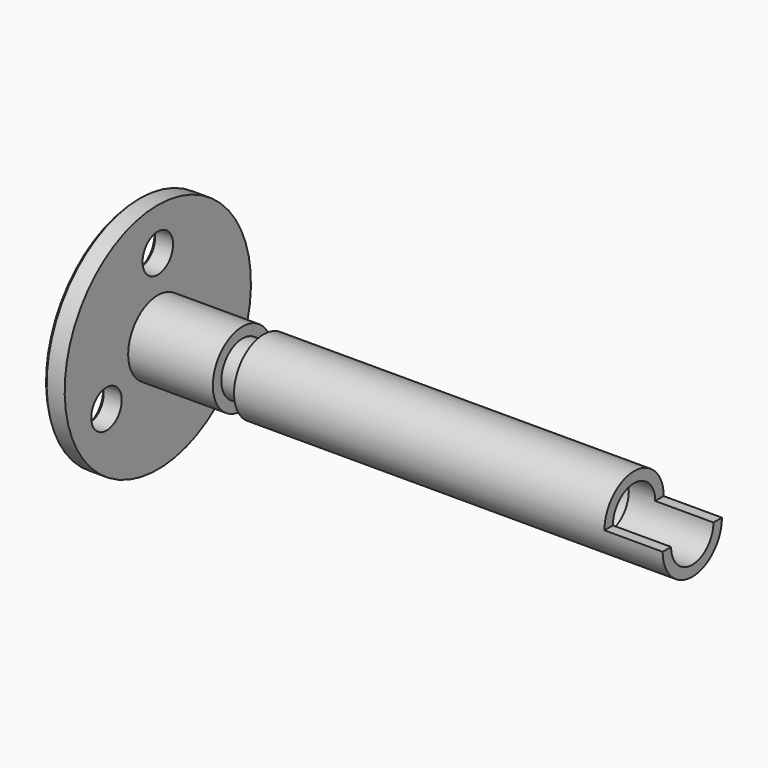
from build123d import *

# Parameters (mm, degrees)
F3_DEPTH        = 5.5
F5_D            = 3.6
F5_COPIES_COUNT = 3
F6_SIZE         = 0.3


# Not quite as in the source:
# - a pattern or mirror of a feature is missing from the dataset's text; its kind, count and spacing are read off the source's solid


with BuildPart() as f1:
    # F0 (on Front) → F1 (revolve)
    with BuildSketch(Plane.XZ):
        Polygon((0, 11), (0, 0), (42, 0), (44.5, 2.5), (52.5, 2.5), (52.5, 3.5), (12, 3.5), (12, 2.5), (10, 2.5), (10, 3.5), (2, 3.5), (2, 11), align=None)
    revolve(axis=Axis((21, 0, 0), (-1, 0, 0)))

    # F2 (on face) → F3 (cut)
    with BuildSketch(Plane.YZ.offset(52.5)):
        with BuildLine():
            Line((2.5, 0), (3.5, 0))
            ThreePointArc((3.5, 0), (0, 3.5), (-3.5, 0))
            Line((-3.5, 0), (-2.5, 0))
            ThreePointArc((-2.5, 0), (0, 2.5), (2.5, 0))
        make_face()
    extrude(amount=-F3_DEPTH, mode=Mode.SUBTRACT)

    # F5 (through all)
    with Locations(Plane(origin=(0, 0, 0), x_dir=(0, -1, 0), z_dir=(-1, 0, 0))):
        with Locations((0, 7)):
            f5 = Hole(F5_D / 2)

    # F5_copies: F5 ×3 about axis
    f5_copies_axis = Axis((0, 0, 0), (1, 0, 0))
    for i in range(1, F5_COPIES_COUNT):
        add(f5.rotate(f5_copies_axis, i * 360 / F5_COPIES_COUNT), mode=Mode.SUBTRACT)

    # F6
    f6_edges = [f1.edges().sort_by_distance(p)[0] for p in [
        (0, 0, -11),
        (0, -6.962178, -1.941154),
        (0, 5.162178, -5.058846),
        (0, 1.8, 7),
    ]]
    chamfer(f6_edges, length=F6_SIZE)


solid = f1.part
